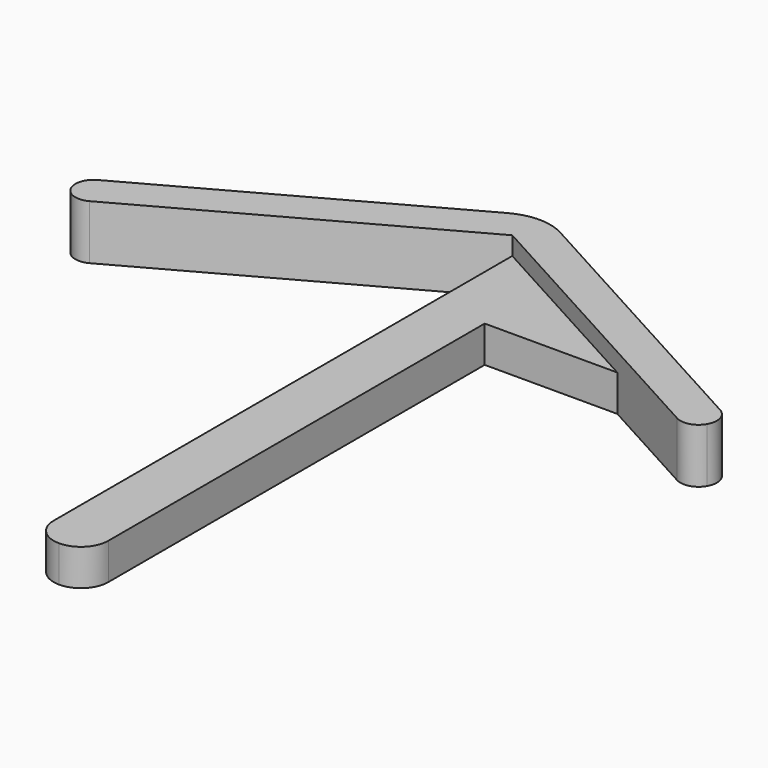
from build123d import *

# Parameters (mm, degrees)
F2_DEPTH      = 15
F3_DEPTH      = 10
F4_R          = 7.49999
F5_R          = 4.99999
F6_R          = 15
F7_W          = 7.5
F7_H          = 2
F8_DEPTH      = 3
F10_TEXT_SIZE = 9.935316947
F15_TEXT_SIZE = 11.1111111111
F11_TEXT_SIZE = 9.6774193548
F12_TEXT_SIZE = 11.1111111111
F13_TEXT_SIZE = 11.1111111111
F14_TEXT_SIZE = 11.1111111111
F16_DEPTH     = 3


# Not quite as in the source:
# - a fillet or chamfer is up to 0.001 mm smaller than in the source, because OpenCascade refuses the exact size
# - Text() gives the source's letters only with a copy of the font that has no kerning and outlines rounded to 1/6400 em; it was checked with that copy


with BuildPart() as f2:
    # F0 (on Top) → F2 (new body)
    with BuildSketch(Plane.XY):
        Polygon((0, 49.3756907964), (-90, 0), (-85, -8.6629683718), (0, 37.9696284915), (85, -8.6629683718), (90, 0), align=None)
    extrude(amount=F2_DEPTH)

    # F1 (on Top) → F3 (join)
    with BuildSketch(Plane.XY):
        Polygon((15, 29.7403466921), (0, 37.9696284915), (0, -127.0303715085), (15, -127.0303715085), (15, 9.7403466921), align=None)
        Polygon((51.4551861648, 9.7403466921), (15, 29.7403466921), (15, 9.7403466921), align=None)
    extrude(amount=F3_DEPTH)

    # F4 (radius 7.5 in the source; OpenCascade refuses exactly that, so slightly less here)
    f4_edges = [f2.edges().sort_by_distance(p)[0] for p in [
        (0, -127.030372, 5),
        (15, -127.030372, 5),
    ]]
    fillet(f4_edges, radius=F4_R)

    # F5 (radius 5 in the source; OpenCascade refuses exactly that, so slightly less here)
    f5_edges = [f2.edges().sort_by_distance(p)[0] for p in [
        (-90, 0, 7.5),
        (-85, -8.662968, 7.5),
        (90, 0, 7.5),
        (85, -8.662968, 7.5),
    ]]
    fillet(f5_edges, radius=F5_R)

    # F6
    f6_edges = [f2.edges().sort_by_distance(p)[0] for p in [
        (0, 49.375691, 7.5),
    ]]
    fillet(f6_edges, radius=F6_R)

    # F7 (on face) → F8 (cut)
    with BuildSketch(Plane(origin=(0, 0, 0), x_dir=(1, 0, 0), z_dir=(0, 0, -1))):
        with Locations((3.75, -12.5696284915)):
            Rectangle(F7_W, F7_H)
        with Locations((3.75, 12.8303715085)):
            Rectangle(F7_W, F7_H)
        with Locations((3.75, 38.2303715085)):
            Rectangle(F7_W, F7_H)
        with Locations((3.75, 63.6303715085)):
            Rectangle(F7_W, F7_H)
        with Locations((3.75, 89.0303715085)):
            Rectangle(F7_W, F7_H)
        with Locations((3.75, 114.4303715085)):
            Rectangle(F7_W, F7_H)
    extrude(amount=-F8_DEPTH, mode=Mode.SUBTRACT)

    # F10 (on face) + F15 (on face) + F11 (on face) + F12 (on face) + F13 (on face) + F14 (on face) → F16 (cut)
    with BuildSketch(Plane(origin=(0, 0, 0), x_dir=(1, 0, 0), z_dir=(0, 0, -1))):
        with Locations((1, 104.2769433067)):
            Text('6', F10_TEXT_SIZE, font='Open Sans', font_style=FontStyle.BOLD, text_align=(TextAlign.LEFT, TextAlign.BOTTOM))
    with BuildSketch(Plane(origin=(0, 0, 0), x_dir=(1, 0, 0), z_dir=(0, 0, -1))):
        with Locations((0.4357638889, 78.0303715085)):
            Text('5', F15_TEXT_SIZE, font='Open Sans', font_style=FontStyle.BOLD, text_align=(TextAlign.LEFT, TextAlign.BOTTOM))
    with BuildSketch(Plane(origin=(0, 0, 0), x_dir=(1, 0, 0), z_dir=(0, 0, -1))):
        with Locations((1, 53.662629573)):
            Text('4', F11_TEXT_SIZE, font='Open Sans', font_style=FontStyle.BOLD, text_align=(TextAlign.LEFT, TextAlign.BOTTOM))
    with BuildSketch(Plane(origin=(0, 0, 0), x_dir=(1, 0, 0), z_dir=(0, 0, -1))):
        with Locations((0.3663194444, 27.2303715085)):
            Text('3', F12_TEXT_SIZE, font='Open Sans', font_style=FontStyle.BOLD, text_align=(TextAlign.LEFT, TextAlign.BOTTOM))
    with BuildSketch(Plane(origin=(0, 0, 0), x_dir=(1, 0, 0), z_dir=(0, 0, -1))):
        with Locations((0.2899305556, 1.8303715085)):
            Text('2', F13_TEXT_SIZE, font='Open Sans', font_style=FontStyle.BOLD, text_align=(TextAlign.LEFT, TextAlign.BOTTOM))
    with BuildSketch(Plane(origin=(0, 0, 0), x_dir=(1, 0, 0), z_dir=(0, 0, -1))):
        with Locations((0.6892361111, -23.5696284915)):
            Text('1', F14_TEXT_SIZE, font='Open Sans', font_style=FontStyle.BOLD, text_align=(TextAlign.LEFT, TextAlign.BOTTOM))
    extrude(amount=-F16_DEPTH, mode=Mode.SUBTRACT)


solid = f2.part
